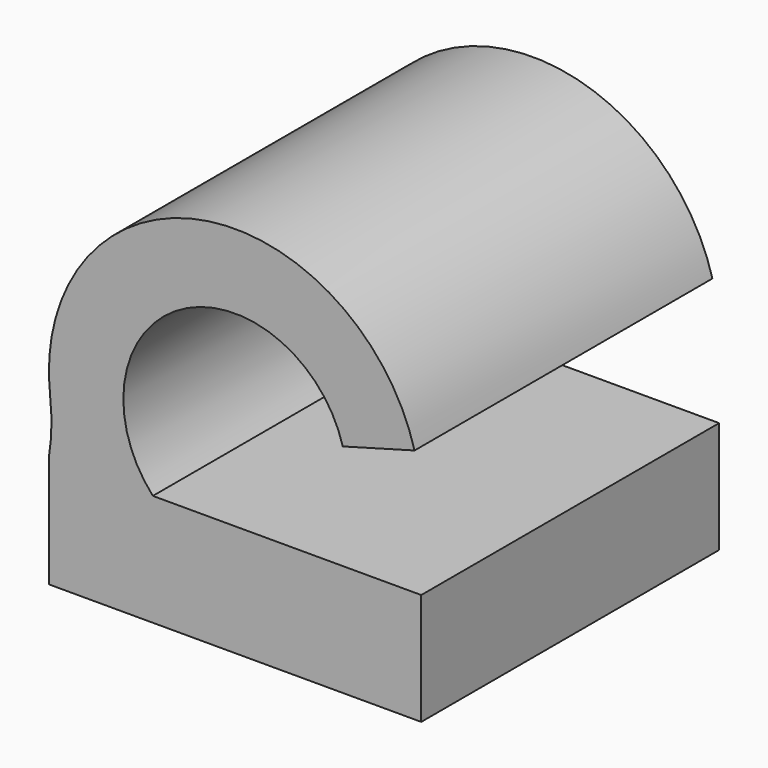
from build123d import *

# Parameters (mm, degrees)
F0_W        = 10
F0_H        = 10
F1_DEPTH    = 3
F3_DEPTH    = 10
F4_T1_DEPTH = 10


# Not quite as in the source:
# - a fillet or chamfer that OpenCascade refuses, or shapes differently, is made with other operations: its cross-section is extruded or revolved along the edge and cut away or added


with BuildPart() as f1:
    # F0 (on Top) → F1 (new body)
    with BuildSketch(Plane.XY):
        Rectangle(F0_W, F0_H)
    extrude(amount=-F1_DEPTH)

    # F2 (on face) → F3 (join)
    with BuildSketch(Plane(origin=(0, 5, 0), x_dir=(-1, 0, 0), z_dir=(0, 1, 0))):
        with BuildLine():
            Line((0, -0.9684120044), (0, -2.9684120044))
            ThreePointArc((0, -2.9684120044), (3.9773759731, 5.0615187488), (-4.8204695111, 3.359395848))
            Line((-4.8204695111, 3.359395848), (-2.8922817066, 2.828272707))
            ThreePointArc((-2.8922817066, 2.828272707), (2.3864255838, 3.8495464475), (0, -0.9684120044))
        make_face()
    extrude(amount=-F3_DEPTH)

    # F4: fillet of radius 5 on 1 edges, made by hand

    # F4_s2 → F4_t1 (join)
    with BuildSketch(Plane.XZ.offset(-5)):
        with BuildLine():
            ThreePointArc((-5, 0), (-4.930361996, 0.7167697097), (-4.9644138164, 1.4361088104))
            ThreePointArc((-4.9644138164, 1.4361088104), (-4.8203188847, 0.7032334307), (-4.5686595645, 0))
            Line((-4.5686595645, 0), (-5, 0))
        make_face()
    extrude(amount=F4_T1_DEPTH)


solid = f1.part
